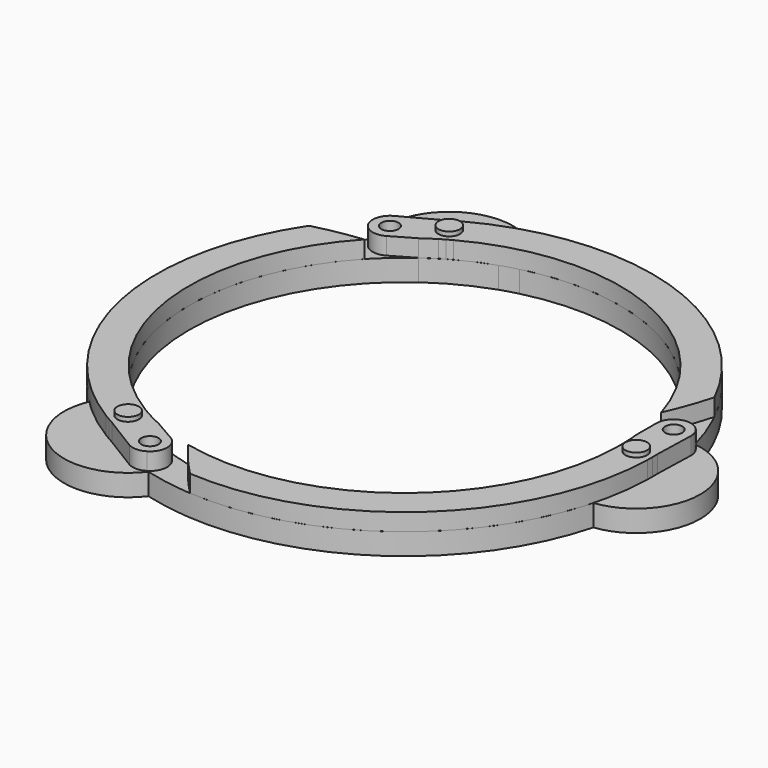
from build123d import *

# Parameters (mm, degrees)
F0_R           = 57.5
F0_R_2         = 50
F1_DEPTH       = 5
F2_R           = 2
F2_R_2         = 2.5
F3_DEPTH       = 4
F5_DEPTH       = 25
F6_R           = 2.5
F7_DEPTH       = 25
F8_COUNT       = 3
F9_R           = 2.5
F10_DEPTH      = 25
F11_R          = 2.5
F12_DEPTH      = 9
F12_DEPTH_BACK = 1
F13_R          = 2.5
F14_DEPTH      = 5


with BuildPart() as f1:
    # F0 (on Top) → F1 (new body)
    with BuildSketch(Plane.XY):
        Circle(F0_R)
        Circle(F0_R_2, mode=Mode.SUBTRACT)
    extrude(amount=F1_DEPTH)

    # F6 (on face) → F7 (cut)
    with BuildSketch(Plane.XY.offset(5)):
        with Locations((53.75, 0)):
            Circle(F6_R)
    extrude(amount=-F7_DEPTH, mode=Mode.SUBTRACT)

    # F9 (on face) → F10 (cut)
    with BuildSketch(Plane.XY.offset(9)):
        with Locations((-26.875, 46.5488654534)):
            Circle(F9_R)
        with Locations((-26.875, -46.5488654534)):
            Circle(F9_R)
    extrude(amount=-F10_DEPTH, mode=Mode.SUBTRACT)

    # F13 (on Top) → F14 (join)
    with BuildSketch(Plane.XY):
        with BuildLine():
            ThreePointArc((-19.1798906539, 54.2068426908), (-17.1125543203, 54.8945396614), (-15.0206493708, 55.503424151))
            ThreePointArc((-15.0206493708, 55.503424151), (-35.0819559672, 58.9325492374), (-39.7409361389, 39.1207137602))
            ThreePointArc((-39.7409361389, 39.1207137602), (-40.140537829, 42.1559899406), (-38.2768345238, 44.5848153754))
            Line((-38.2768345238, 44.5848153754), (-37.6120013916, 44.9438345083))
            ThreePointArc((-37.6120013916, 44.9438345083), (-31.7498443002, 56.2491343294), (-19.1798906539, 54.2068426908))
        make_face()
        with BuildLine():
            ThreePointArc((-29.9876888917, 49.0610692396), (-24.7180595051, 51.9159660827), (-19.1798906539, 54.2068426908))
            ThreePointArc((-19.1798906539, 54.2068426908), (-31.7498443002, 56.2491343294), (-37.6120013916, 44.9438345083))
            Line((-37.6120013916, 44.9438345083), (-29.9876888917, 49.0610692396))
        make_face()
        with BuildLine():
            ThreePointArc((-38.2768345238, 44.5848153754), (-40.140537829, 42.1559899406), (-39.7409361389, 39.1207137602))
            ThreePointArc((-39.7409361389, 39.1207137602), (-37.3121107042, 37.2570104551), (-34.2768345238, 37.6566121451))
            Line((-34.2768345238, 37.6566121451), (-33.6153942939, 38.0384948399))
            ThreePointArc((-33.6153942939, 38.0384948399), (-36.2710507114, 41.1107082061), (-37.6120013916, 44.9438345083))
            Line((-37.6120013916, 44.9438345083), (-38.2768345238, 44.5848153754))
        make_face()
        with BuildLine():
            ThreePointArc((-16.0486249897, 47.3544257271), (-17.0007784989, 51.0609683961), (-19.1798906539, 54.2068426908))
            ThreePointArc((-19.1798906539, 54.2068426908), (-24.7180595051, 51.9159660827), (-29.9876888917, 49.0610692396))
            Line((-29.9876888917, 49.0610692396), (-37.6120013916, 44.9438345083))
            ThreePointArc((-37.6120013916, 44.9438345083), (-36.2710507114, 41.1107082061), (-33.6153942939, 38.0384948399))
            Line((-33.6153942939, 38.0384948399), (-29.199710973, 40.5878907938))
            ThreePointArc((-29.199710973, 40.5878907938), (-22.8757398919, 44.4601003643), (-16.0486249897, 47.3544257271))
        make_face()
        with Locations((-26.875, 46.5488654534)):
            Circle(F13_R, mode=Mode.SUBTRACT)
        with BuildLine():
            ThreePointArc((-27.4942878525, -50.5006350008), (-32.6015157371, -47.364450505), (-37.3545575023, -43.7136938935))
            ThreePointArc((-37.3545575023, -43.7136938935), (-32.83825712, -55.6207388949), (-20.1165017318, -55.0448659464))
            Line((-20.1165017318, -55.0448659464), (-27.4942878525, -50.5006350008))
        make_face()
        with BuildLine():
            ThreePointArc((-37.3545575023, -43.7136938935), (-38.9837887157, -42.2671765957), (-40.5570506264, -40.7599760119))
            ThreePointArc((-40.5570506264, -40.7599760119), (-33.4961067657, -59.8481397007), (-14.0090638611, -53.9770171466))
            ThreePointArc((-14.0090638611, -53.9770171466), (-16.4378892958, -55.8407204518), (-19.4731654762, -55.4411187617))
            Line((-19.4731654762, -55.4411187617), (-20.1165017318, -55.0448659464))
            ThreePointArc((-20.1165017318, -55.0448659464), (-32.83825712, -55.6207388949), (-37.3545575023, -43.7136938935))
        make_face()
        with BuildLine():
            ThreePointArc((-19.4731654762, -55.4411187617), (-16.4378892958, -55.8407204518), (-14.0090638611, -53.9770171466))
            ThreePointArc((-14.0090638611, -53.9770171466), (-13.609462171, -50.9417409662), (-15.4731654762, -48.5129155315))
            Line((-15.4731654762, -48.5129155315), (-16.1346057061, -48.1310328367))
            ThreePointArc((-16.1346057061, -48.1310328367), (-17.4673923183, -51.967005441), (-20.1165017318, -55.0448659464))
            Line((-20.1165017318, -55.0448659464), (-19.4731654762, -55.4411187617))
        make_face()
        with BuildLine():
            ThreePointArc((-32.9858231664, -37.5757298004), (-35.7197065234, -40.2535902622), (-37.3545575023, -43.7136938935))
            ThreePointArc((-37.3545575023, -43.7136938935), (-32.6015157371, -47.364450505), (-27.4942878525, -50.5006350008))
            Line((-27.4942878525, -50.5006350008), (-20.1165017318, -55.0448659464))
            ThreePointArc((-20.1165017318, -55.0448659464), (-17.4673923183, -51.967005441), (-16.1346057061, -48.1310328367))
            Line((-16.1346057061, -48.1310328367), (-20.550289027, -45.5816368827))
            ThreePointArc((-20.550289027, -45.5816368827), (-27.0657064243, -42.0410220588), (-32.9858231664, -37.5757298004))
        make_face()
        with Locations((-26.875, -46.5488654534)):
            Circle(F13_R, mode=Mode.SUBTRACT)
        with BuildLine():
            ThreePointArc((57.4819767442, 1.4395657612), (57.3195752422, -4.5515155777), (56.5344481561, -10.4931487973))
            ThreePointArc((56.5344481561, -10.4931487973), (64.5881014202, -0.6283954345), (57.7285031234, 10.1010314381))
            Line((57.7285031234, 10.1010314381), (57.4819767442, 1.4395657612))
        make_face()
        with BuildLine():
            ThreePointArc((56.5344481561, -10.4931487973), (56.096343036, -12.6273630657), (55.5776999971, -14.7434481391))
            ThreePointArc((55.5776999971, -14.7434481391), (68.5780627329, 0.9155904634), (53.75, 14.8563033864))
            ThreePointArc((53.75, 14.8563033864), (56.5784271247, 13.6847305111), (57.75, 10.8563033864))
            Line((57.75, 10.8563033864), (57.7285031234, 10.1010314381))
            ThreePointArc((57.7285031234, 10.1010314381), (64.5881014202, -0.6283954345), (56.5344481561, -10.4931487973))
        make_face()
        with BuildLine():
            ThreePointArc((57.75, 10.8563033864), (56.5784271247, 13.6847305111), (53.75, 14.8563033864))
            ThreePointArc((53.75, 14.8563033864), (50.9215728753, 13.6847305111), (49.75, 10.8563033864))
            Line((49.75, 10.8563033864), (49.75, 10.0925379968))
            ThreePointArc((49.75, 10.0925379968), (53.7384430297, 10.856297235), (57.7285031234, 10.1010314381))
            Line((57.7285031234, 10.1010314381), (57.75, 10.8563033864))
        make_face()
        with BuildLine():
            ThreePointArc((49.0344481561, -9.7786959266), (52.7204850223, -10.8073781338), (56.5344481561, -10.4931487973))
            ThreePointArc((56.5344481561, -10.4931487973), (57.3195752422, -4.5515155777), (57.4819767442, 1.4395657612))
            Line((57.4819767442, 1.4395657612), (57.7285031234, 10.1010314381))
            ThreePointArc((57.7285031234, 10.1010314381), (53.7384430297, 10.856297235), (49.75, 10.0925379968))
            Line((49.75, 10.0925379968), (49.75, 4.9937460889))
            ThreePointArc((49.75, 4.9937460889), (49.9414463162, -2.4190783054), (49.0344481561, -9.7786959266))
        make_face()
        with Locations((53.75, 0)):
            Circle(F13_R, mode=Mode.SUBTRACT)
        with BuildLine():
            ThreePointArc((48.0776999971, -13.7307961527), (51.7621359925, -14.7227085482), (55.5776999971, -14.7434481391))
            ThreePointArc((55.5776999971, -14.7434481391), (56.096343036, -12.6273630657), (56.5344481561, -10.4931487973))
            ThreePointArc((56.5344481561, -10.4931487973), (52.7204850223, -10.8073781338), (49.0344481561, -9.7786959266))
            ThreePointArc((49.0344481561, -9.7786959266), (48.5962663564, -11.7644760281), (48.0776999971, -13.7307961527))
        make_face()
        with BuildLine():
            ThreePointArc((-12.1476317162, 48.5019076294), (-13.130828381, 52.1886789977), (-15.0206493708, 55.503424151))
            ThreePointArc((-15.0206493708, 55.503424151), (-17.1125543203, 54.8945396614), (-19.1798906539, 54.2068426908))
            ThreePointArc((-19.1798906539, 54.2068426908), (-17.0007784989, 51.0609683961), (-16.0486249897, 47.3544257271))
            ThreePointArc((-16.0486249897, 47.3544257271), (-14.1097980756, 47.9678392078), (-12.1476317162, 48.5019076294))
        make_face()
    extrude(amount=F14_DEPTH)


with BuildPart() as f3:
    # F2 (on face) → F3 (new body)
    with BuildSketch(Plane.XY.offset(5)):
        with BuildLine():
            Line((57.75, 0), (57.75, 10.8563033864))
            ThreePointArc((57.75, 10.8563033864), (57.5280684467, 9.5424545321), (56.8869005941, 8.3743979364))
            ThreePointArc((56.8869005941, 8.3743979364), (57.2894667476, 4.915994281), (57.4819767442, 1.4395657612))
            ThreePointArc((57.4819767442, 1.4395657612), (57.6824233608, 0.732151973), (57.75, 0))
        make_face()
        with BuildLine():
            Line((49.75, 10.8563033864), (49.75, 4.9937460889))
            ThreePointArc((49.75, 4.9937460889), (49.8993978277, 3.170188707), (49.9819767442, 1.3423862126))
            ThreePointArc((49.9819767442, 1.3423862126), (53.6981752577, 3.9996642604), (57.4819767442, 1.4395657612))
            ThreePointArc((57.4819767442, 1.4395657612), (57.2894667476, 4.915994281), (56.8869005941, 8.3743979364))
            ThreePointArc((56.8869005941, 8.3743979364), (52.4361511458, 7.0782349397), (49.75, 10.8563033864))
        make_face()
        with BuildLine():
            ThreePointArc((56.8869005941, 8.3743979364), (56.3618506441, 11.38383907), (55.6777104591, 14.3611475178))
            ThreePointArc((55.6777104591, 14.3611475178), (51.7141760681, 14.2994735707), (49.75, 10.8563033864))
            ThreePointArc((49.75, 10.8563033864), (52.4361511458, 7.0782349397), (56.8869005941, 8.3743979364))
        make_face()
        with Locations((53.75, 10.8563033864)):
            Circle(F2_R, mode=Mode.SUBTRACT)
        with BuildLine():
            ThreePointArc((57.75, 10.8563033864), (57.1931701843, 12.8921273183), (55.6777104591, 14.3611475178))
            ThreePointArc((55.6777104591, 14.3611475178), (56.3618506441, 11.38383907), (56.8869005941, 8.3743979364))
            ThreePointArc((56.8869005941, 8.3743979364), (57.5280684467, 9.5424545321), (57.75, 10.8563033864))
        make_face()
        with BuildLine():
            ThreePointArc((57.4819767442, 1.4395657612), (53.6981752577, 3.9996642604), (49.9819767442, 1.3423862126))
            ThreePointArc((49.9819767442, 1.3423862126), (49.995493983, 0.6712535999), (50, 0))
            ThreePointArc((50, 0), (49.995493983, -0.6712535999), (49.9819767442, -1.3423862126))
            ThreePointArc((49.9819767442, -1.3423862126), (53.6981752577, -3.9996642604), (57.4819767442, -1.4395657612))
            ThreePointArc((57.4819767442, -1.4395657612), (57.4954940095, -0.7198392908), (57.5, 0))
            ThreePointArc((57.5, 0), (57.4954940095, 0.7198392908), (57.4819767442, 1.4395657612))
        make_face()
        with Locations((53.75, 0)):
            Circle(F2_R_2, mode=Mode.SUBTRACT)
        with BuildLine():
            ThreePointArc((57.4819767442, -1.4395657612), (53.6981752577, -3.9996642604), (49.9819767442, -1.3423862126))
            ThreePointArc((49.9819767442, -1.3423862126), (30.6127445505, -39.5330225392), (-11.2102238263, -48.7271062322))
            ThreePointArc((-11.2102238263, -48.7271062322), (-7.6890307836, -53.1779496641), (-3.86345578, -57.3700593466))
            ThreePointArc((-3.86345578, -57.3700593466), (38.7400500229, -42.4906875), (57.4819767442, -1.4395657612))
        make_face()
    extrude(amount=F3_DEPTH)

    # F4 (on face) → F5 (cut)
    with BuildSketch(Plane.XY.offset(9)):
        with BuildLine():
            Line((57.75, 10.8563033864), (57.4819767442, 1.4395657612))
            ThreePointArc((57.4819767442, 1.4395657612), (57.6824233608, 0.732151973), (57.75, 0))
            Line((57.75, 0), (57.75, 10.8563033864))
        make_face()
        with BuildLine():
            ThreePointArc((57.4819767442, 1.4395657612), (57.4967126165, 0.6148481892), (57.4996165354, -0.2099959092))
            Line((57.4996165354, -0.2099959092), (59.8347745836, -1.3514566235))
            Line((59.8347745836, -1.3514566235), (61.8689011848, 10.7390694408))
            Line((61.8689011848, 10.7390694408), (57.75, 10.8563033864))
            Line((57.75, 10.8563033864), (57.75, 0))
            ThreePointArc((57.75, 0), (57.6824233608, 0.732151973), (57.4819767442, 1.4395657612))
        make_face()
    extrude(amount=-F5_DEPTH, mode=Mode.SUBTRACT)


with BuildPart() as f8_1:
    # F8: instance of F3
    add(f3.part.rotate(Axis((0, 0, 0), (0, 0, 1)), 1 * 360 / F8_COUNT))


with BuildPart() as f8_2:
    # F8: instance of F3
    add(f3.part.rotate(Axis((0, 0, 0), (0, 0, 1)), 2 * 360 / F8_COUNT))


with BuildPart() as f12:
    # F11 (on face) → F12 (new body, two sides)
    with BuildSketch(Plane.XY.offset(9)) as f12_sk:
        with Locations((-26.875, 46.5488654534)):
            Circle(F11_R)
    extrude(amount=-F12_DEPTH)
    extrude(f12_sk.sketch, amount=F12_DEPTH_BACK)


with BuildPart() as f12b:
    # F11 (on face) → F12, piece 2 (new body, two sides)
    with BuildSketch(Plane.XY.offset(9)) as f12_2_sk:
        with Locations((53.75, 0)):
            Circle(F11_R)
    extrude(amount=-F12_DEPTH)
    extrude(f12_2_sk.sketch, amount=F12_DEPTH_BACK)


with BuildPart() as f12c:
    # F11 (on face) → F12, piece 3 (new body, two sides)
    with BuildSketch(Plane.XY.offset(9)) as f12_3_sk:
        with Locations((-26.875, -46.5488654534)):
            Circle(F11_R)
    extrude(amount=-F12_DEPTH)
    extrude(f12_3_sk.sketch, amount=F12_DEPTH_BACK)


solid = Compound([f1.part, f3.part, f8_1.part, f8_2.part, f12.part, f12b.part, f12c.part])
